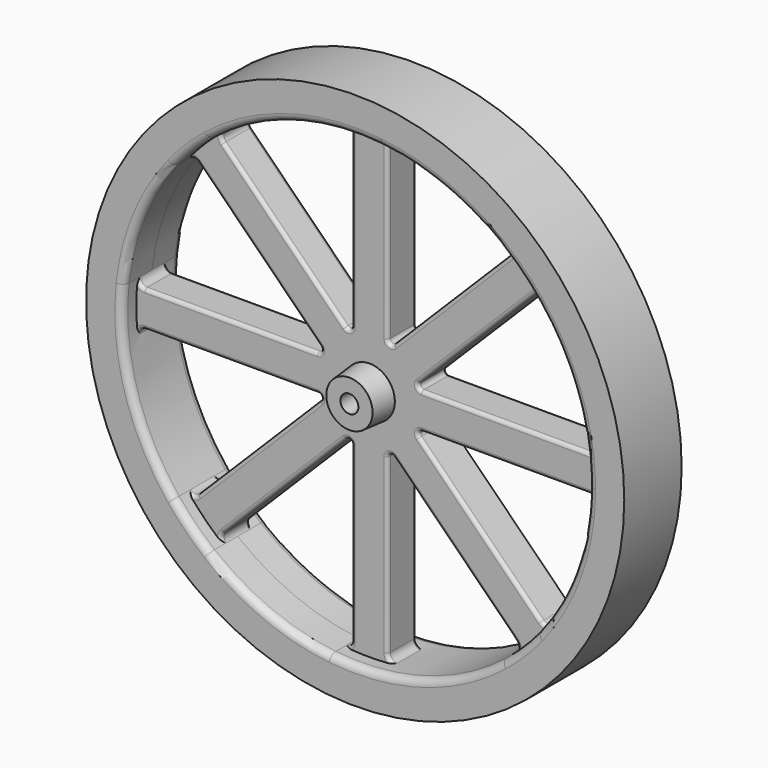
from build123d import *

# Parameters (mm, degrees)
F0_R     = 75
F1_DEPTH = 10
F0_R_2   = 7.5
F0_R_3   = 2.5
F2_DEPTH = 5
F3_DEPTH = 12
F3_TAPER = 5
F4_DEPTH = 12.5
F5_R     = 2
F6_R     = 1


with BuildPart() as f1:
    # F0 (on Front) → F1 (new body, symmetric)
    with BuildSketch(Plane.XZ):
        Circle(F0_R)
        with BuildLine():
            ThreePointArc((-50.6443861035, 40.7448911669), (-45.9619407771, 45.9619407771), (-40.7448911669, 50.6443861035))
            ThreePointArc((-40.7448911669, 50.6443861035), (-24.8744231037, 60.0521696132), (-7, 64.6219776856))
            ThreePointArc((-7, 64.6219776856), (0, 65), (7, 64.6219776856))
            ThreePointArc((7, 64.6219776856), (24.8744231037, 60.0521696132), (40.7448911669, 50.6443861035))
            ThreePointArc((40.7448911669, 50.6443861035), (45.9619407771, 45.9619407771), (50.6443861035, 40.7448911669))
            ThreePointArc((50.6443861035, 40.7448911669), (60.0521696132, 24.8744231037), (64.6219776856, 7))
            ThreePointArc((64.6219776856, 7), (64.905425619, 3.505099887), (65, 0))
            ThreePointArc((65, 0), (64.905425619, -3.505099887), (64.6219776856, -7))
            ThreePointArc((64.6219776856, -7), (60.0521696132, -24.8744231037), (50.6443861035, -40.7448911669))
            ThreePointArc((50.6443861035, -40.7448911669), (45.9619407771, -45.9619407771), (40.7448911669, -50.6443861035))
            ThreePointArc((40.7448911669, -50.6443861035), (24.8744231037, -60.0521696132), (7, -64.6219776856))
            ThreePointArc((7, -64.6219776856), (0, -65), (-7, -64.6219776856))
            ThreePointArc((-7, -64.6219776856), (-24.8744231037, -60.0521696132), (-40.7448911669, -50.6443861035))
            ThreePointArc((-40.7448911669, -50.6443861035), (-45.9619407771, -45.9619407771), (-50.6443861035, -40.7448911669))
            ThreePointArc((-50.6443861035, -40.7448911669), (-60.0521696132, -24.8744231037), (-64.6219776856, -7))
            ThreePointArc((-64.6219776856, -7), (-65, 0), (-64.6219776856, 7))
            ThreePointArc((-64.6219776856, 7), (-60.0521696132, 24.8744231037), (-50.6443861035, 40.7448911669))
        make_face(mode=Mode.SUBTRACT)
    extrude(amount=F1_DEPTH, both=True)

    # F0 (on Front) → F2 (join, symmetric)
    with BuildSketch(Plane.XZ):
        with BuildLine():
            ThreePointArc((-5, 14.4852813742), (-5.6173165676, 13.5614018417), (-6.7071067812, 13.7781745931))
            Line((-6.7071067812, 13.7781745931), (-40.7448911669, 47.8159589787))
            ThreePointArc((-40.7448911669, 47.8159589787), (-41.3306776045, 49.2301725411), (-40.7448911669, 50.6443861035))
            ThreePointArc((-40.7448911669, 50.6443861035), (-45.9619407771, 45.9619407771), (-50.6443861035, 40.7448911669))
            ThreePointArc((-50.6443861035, 40.7448911669), (-49.2301725411, 41.3306776045), (-47.8159589787, 40.7448911669))
            Line((-47.8159589787, 40.7448911669), (-13.7781745931, 6.7071067812))
            ThreePointArc((-13.7781745931, 6.7071067812), (-13.5614018417, 5.6173165676), (-14.4852813742, 5))
            Line((-14.4852813742, 5), (-62.6219776856, 5))
            ThreePointArc((-62.6219776856, 5), (-64.036191248, 5.5857864376), (-64.6219776856, 7))
            ThreePointArc((-64.6219776856, 7), (-65, 0), (-64.6219776856, -7))
            ThreePointArc((-64.6219776856, -7), (-64.036191248, -5.5857864376), (-62.6219776856, -5))
            Line((-62.6219776856, -5), (-14.4852813742, -5))
            ThreePointArc((-14.4852813742, -5), (-13.5614018417, -5.6173165676), (-13.7781745931, -6.7071067812))
            Line((-13.7781745931, -6.7071067812), (-47.8159589787, -40.7448911669))
            ThreePointArc((-47.8159589787, -40.7448911669), (-49.2301725411, -41.3306776045), (-50.6443861035, -40.7448911669))
            ThreePointArc((-50.6443861035, -40.7448911669), (-45.9619407771, -45.9619407771), (-40.7448911669, -50.6443861035))
            ThreePointArc((-40.7448911669, -50.6443861035), (-41.3306776045, -49.2301725411), (-40.7448911669, -47.8159589787))
            Line((-40.7448911669, -47.8159589787), (-6.7071067812, -13.7781745931))
            ThreePointArc((-6.7071067812, -13.7781745931), (-5.6173165676, -13.5614018417), (-5, -14.4852813742))
            Line((-5, -14.4852813742), (-5, -62.6219776856))
            ThreePointArc((-5, -62.6219776856), (-5.5857864376, -64.036191248), (-7, -64.6219776856))
            ThreePointArc((-7, -64.6219776856), (0, -65), (7, -64.6219776856))
            ThreePointArc((7, -64.6219776856), (5.5857864376, -64.036191248), (5, -62.6219776856))
            Line((5, -62.6219776856), (5, -14.4852813742))
            ThreePointArc((5, -14.4852813742), (5.6173165676, -13.5614018417), (6.7071067812, -13.7781745931))
            Line((6.7071067812, -13.7781745931), (40.7448911669, -47.8159589787))
            ThreePointArc((40.7448911669, -47.8159589787), (41.3306776045, -49.2301725411), (40.7448911669, -50.6443861035))
            ThreePointArc((40.7448911669, -50.6443861035), (45.9619407771, -45.9619407771), (50.6443861035, -40.7448911669))
            ThreePointArc((50.6443861035, -40.7448911669), (49.2301725411, -41.3306776045), (47.8159589787, -40.7448911669))
            Line((47.8159589787, -40.7448911669), (13.7781745931, -6.7071067812))
            ThreePointArc((13.7781745931, -6.7071067812), (13.5614018417, -5.6173165676), (14.4852813742, -5))
            Line((14.4852813742, -5), (62.6219776856, -5))
            ThreePointArc((62.6219776856, -5), (64.036191248, -5.5857864376), (64.6219776856, -7))
            ThreePointArc((64.6219776856, -7), (64.905425619, -3.505099887), (65, 0))
            ThreePointArc((65, 0), (64.905425619, 3.505099887), (64.6219776856, 7))
            ThreePointArc((64.6219776856, 7), (64.036191248, 5.5857864376), (62.6219776856, 5))
            Line((62.6219776856, 5), (14.4852813742, 5))
            ThreePointArc((14.4852813742, 5), (13.5614018417, 5.6173165676), (13.7781745931, 6.7071067812))
            Line((13.7781745931, 6.7071067812), (47.8159589787, 40.7448911669))
            ThreePointArc((47.8159589787, 40.7448911669), (49.2301725411, 41.3306776045), (50.6443861035, 40.7448911669))
            ThreePointArc((50.6443861035, 40.7448911669), (45.9619407771, 45.9619407771), (40.7448911669, 50.6443861035))
            ThreePointArc((40.7448911669, 50.6443861035), (41.3306776045, 49.2301725411), (40.7448911669, 47.8159589787))
            Line((40.7448911669, 47.8159589787), (6.7071067812, 13.7781745931))
            ThreePointArc((6.7071067812, 13.7781745931), (5.6173165676, 13.5614018417), (5, 14.4852813742))
            Line((5, 14.4852813742), (5, 62.6219776856))
            ThreePointArc((5, 62.6219776856), (5.5857864376, 64.036191248), (7, 64.6219776856))
            ThreePointArc((7, 64.6219776856), (0, 65), (-7, 64.6219776856))
            ThreePointArc((-7, 64.6219776856), (-5.5857864376, 64.036191248), (-5, 62.6219776856))
            Line((-5, 62.6219776856), (-5, 14.4852813742))
        make_face()
        Circle(F0_R_2, mode=Mode.SUBTRACT)
        Circle(F0_R_2)
        Circle(F0_R_3, mode=Mode.SUBTRACT)
    extrude(amount=F2_DEPTH, both=True)

    # F0 (on Front) → F3 (join, symmetric)
    with BuildSketch(Plane.XZ):
        Circle(F0_R_2)
        Circle(F0_R_3, mode=Mode.SUBTRACT)
        Circle(F0_R_3)
    extrude(amount=F3_DEPTH, both=True, taper=F3_TAPER)

    # F0 (on Front) → F4 (cut, symmetric)
    with BuildSketch(Plane.XZ):
        Circle(F0_R_3)
    extrude(amount=F4_DEPTH, both=True, mode=Mode.SUBTRACT)

    # F5
    f5_edges = [f1.edges().sort_by_distance(p)[0] for p in [
        (-65, 10, 0),
        (-65, -10, 0),
    ]]
    fillet(f5_edges, radius=F5_R)

    # F6
    f6_edges = [f1.edges().sort_by_distance(p)[0] for p in [
        (-30.797067, -5, 23.725999),
        (-38.55363, -5, -5),
        (-23.725999, -5, -30.797067),
        (5, -5, -38.55363),
        (30.797067, -5, -23.725999),
        (38.55363, -5, 5),
        (23.725999, -5, 30.797067),
        (-5, -5, 38.55363),
        (-38.55363, 5, -5),
        (-23.725999, 5, -30.797067),
        (-5, 5, 38.55363),
        (23.725999, 5, 30.797067),
        (38.55363, 5, 5),
        (-30.797067, 5, 23.725999),
        (5, 5, -38.55363),
    ]]
    fillet(f6_edges, radius=F6_R)


solid = f1.part
